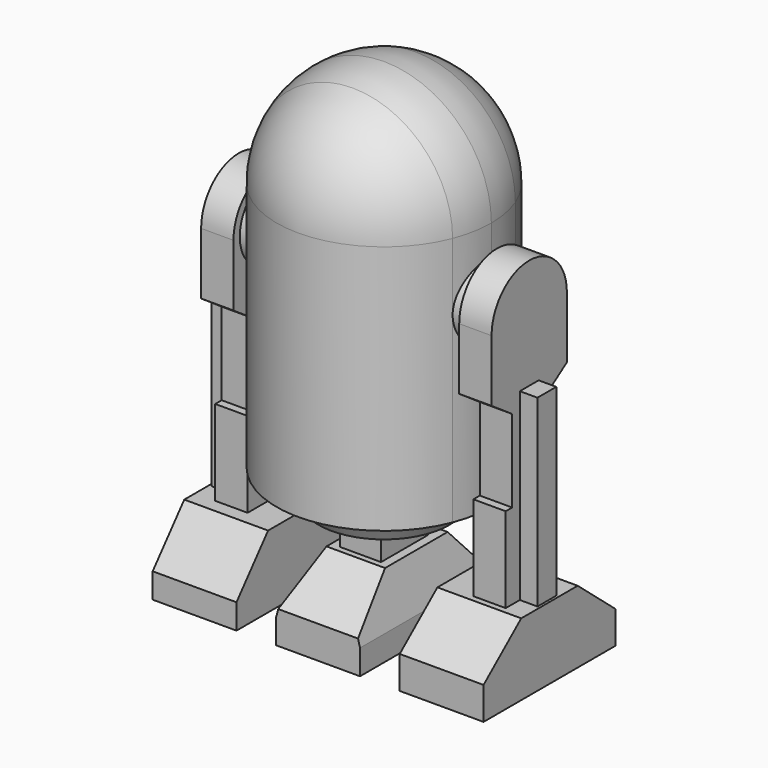
from build123d import *

# Parameters (mm, degrees)
F1_DEPTH       = 539.75
F2_ANGLE       = 180
F3_START       = -146.05
F3_DEPTH       = 568.325
F4_W           = 69.85
F4_H           = 101.6
F7_DEPTH       = 69.85
F8_W           = 50.8
F8_H           = 431.8
F9_DEPTH       = 38.1
F6_R           = 84.582
F11_DEPTH      = 627.0625
F12_R          = 177.8
F13_DEPTH      = 63.5
F14_SIZE2      = 36.661732
F14_SIZE       = 63.49999
F16_W          = 180.975
F16_H          = 355.6
F17_DEPTH      = 155.575
F18_W          = 88.9
F18_H          = 127
F19_DEPTH      = 76.2
F20_C1_SIZE2   = 85.2525225276
F20_C1_SIZE    = 101.6
F20_C2_SIZE2   = 85.2525225276
F20_C2_SIZE    = 101.6
F20_C3_SIZE2   = 85.2525225276
F20_C3_SIZE    = 101.6
F20_C4_SIZE2   = 85.2525225276
F20_C4_SIZE    = 101.6
F20_C5_SIZE2   = 101.6
F20_C5_SIZE    = 85.2525225276
F20_C6_SIZE2   = 85.2525225276
F20_C6_SIZE    = 101.6
F21_SIZE2      = 27.223637951
F21_SIZE       = 101.6
F21_2_SIZE2    = 27.223637951
F21_2_SIZE     = 101.6
F23_DEPTH      = 1136.65
F23_DEPTH_BACK = 101.6
F22_W          = 6.35
F22_H          = 457.2
F22_W_2        = 736.6
F22_H_2        = 6.35
F24_DEPTH      = 12.7
F25_DEPTH      = 1136.65
F26_W          = 38.1
F26_H          = 88.9
F27_DEPTH      = 457.2
F29_W          = 38.1
F29_H          = 63.5
F30_DEPTH      = 6.35
F31_W          = 38.1
F31_H          = 63.5
F32_DEPTH      = 12.7
F31_W_2        = 812.8
F31_H_2        = 114.3
F33_W          = 38.1
F33_H          = 584.2
F34_DEPTH      = 88.9
F35_W          = 38.1
F35_H          = 63.5
F36_DEPTH      = 736.6


# Not quite as in the source:
# - a fillet or chamfer is up to 0.001 mm smaller than in the source, because OpenCascade refuses the exact size
# - a feature of the source that left no trace in its solid (it failed there, or was rolled back) is left out


with BuildPart() as f1:
    # F0 (on Top) → F1 (new body)
    with BuildSketch(Plane.XY):
        with BuildLine():
            ThreePointArc((215.7904907567, -84.582), (227.743816184, -43.0395726621), (231.775, 0))
            ThreePointArc((231.775, 0), (227.743816184, 43.0395726621), (215.7904907567, 84.582))
            ThreePointArc((215.7904907567, 84.582), (130.6056231083, 191.4727704858), (0, 231.775))
            Line((0, 231.775), (0, 0))
            Line((0, 0), (0, -231.775))
            ThreePointArc((0, -231.775), (130.6056231083, -191.4727704858), (215.7904907567, -84.582))
        make_face()
        with BuildLine():
            Line((0, 0), (0, 231.775))
            ThreePointArc((0, 231.775), (-130.6056231083, 191.4727704858), (-215.7904907567, 84.582))
            ThreePointArc((-215.7904907567, 84.582), (-231.775, 0), (-215.7904907567, -84.582))
            ThreePointArc((-215.7904907567, -84.582), (-130.6056231083, -191.4727704858), (0, -231.775))
            Line((0, -231.775), (0, 0))
        make_face()
    extrude(amount=-F1_DEPTH)

    # F0 (on Top) → F2 (revolve)
    with BuildSketch(Plane.XY):
        with BuildLine():
            ThreePointArc((215.7904907567, -84.582), (227.743816184, -43.0395726621), (231.775, 0))
            ThreePointArc((231.775, 0), (227.743816184, 43.0395726621), (215.7904907567, 84.582))
            ThreePointArc((215.7904907567, 84.582), (130.6056231083, 191.4727704858), (0, 231.775))
            Line((0, 231.775), (0, 0))
            Line((0, 0), (0, -231.775))
            ThreePointArc((0, -231.775), (130.6056231083, -191.4727704858), (215.7904907567, -84.582))
        make_face()
    revolve(axis=Axis((0, -115.8875, 0), (0, -1, 0)), revolution_arc=F2_ANGLE)



with BuildPart() as f3:
    # F0 (on Top) → F3 (new body)
    with BuildSketch(Plane.XY.offset(F3_START)):
        Polygon((243.68125, 0), (243.68125, -84.582), (243.68125, -101.6), (313.53125, -101.6), (313.53125, -50.8), (313.53125, 0), align=None)
        Polygon((243.68125, 101.6), (243.68125, 84.582), (243.68125, 0), (313.53125, 0), (313.53125, 50.8), (313.53125, 101.6), align=None)
    extrude(amount=-F3_DEPTH)

    # F4 (on face) → F5 (revolve)
    with BuildSketch(Plane.XY.offset(-146.05)):
        with Locations((278.60625, -50.8)):
            Rectangle(F4_W, F4_H)
    revolve(axis=Axis((278.60625, 0, -146.05), (-1, 0, 0)))

    # F6 (on face) → F7 (cut, through all)
    with BuildSketch(Plane.YZ.offset(313.53125)):
        Polygon((101.6, -279.4), (46.0375, -317.5), (46.0375, -495.3), (63.5, -495.3), (63.5, -714.375), (101.6, -714.375), align=None)
        Polygon((-101.6, -714.375), (-63.5, -714.375), (-63.5, -495.3), (-46.0375, -495.3), (-46.0375, -317.5), (-101.6, -279.4), align=None)
    extrude(amount=-F7_DEPTH, mode=Mode.SUBTRACT)

    # F8 (on face) → F9 (join)
    with BuildSketch(Plane.YZ.offset(313.53125)):
        with Locations((0, -498.475)):
            Rectangle(F8_W, F8_H)
    extrude(amount=F9_DEPTH)


with BuildPart() as f10_1:
    # F10: instance of F3
    add(f3.part.mirror(Plane.YZ))


with BuildPart() as f1_1:
    add(f1.part)

    add(f3.part)  # F11 merges F3

    add(f10_1.part)  # F11 merges F10_1
    # F6 (on face) → F11 (join, through all)
    with BuildSketch(Plane.YZ.offset(313.53125)):
        with Locations((0, -146.05)):
            Circle(F6_R)
    extrude(amount=-F11_DEPTH)

    # F12 (on face) → F13 (join)
    with BuildSketch(Plane(origin=(0, 0, -539.75), x_dir=(1, 0, 0), z_dir=(0, 0, -1))):
        Circle(F12_R)
    extrude(amount=F13_DEPTH)

    # F14 (size 63.5 and 36.6617420935 in the source; OpenCascade refuses exactly that, so slightly less here)
    f14_edges = [f1_1.edges().sort_by_distance(p)[0] for p in [
        (-177.8, 0, -603.25),
    ]]
    f14_side = f1_1.faces().sort_by_distance((-177.8, 0, -571.5))[0]
    chamfer(f14_edges, length=F14_SIZE, length2=F14_SIZE2, reference=f14_side)

    # F16 (on offset) → F17, piece 2 (join)
    with BuildSketch(Plane.XY.offset(-835.025)):
        with Locations((-266.7, 0)):
            Rectangle(F16_W, F16_H)
        with Locations((266.7, 0)):
            Rectangle(F16_W, F16_H)
    extrude(amount=F17_DEPTH)



with BuildPart() as f17:
    # F16 (on offset) → F17 (new body)
    with BuildSketch(Plane.XY.offset(-835.025)):
        Rectangle(F16_W, F16_H)
    extrude(amount=F17_DEPTH)


with BuildPart() as f1_2:
    add(f1_1.part)

    add(f17.part)  # F19 merges F17
    # F18 (on face) → F19 (join, through all)
    with BuildSketch(Plane.XY.offset(-679.45)):
        Rectangle(F18_W, F18_H)
    extrude(amount=F19_DEPTH)

    # F20: chamfer of 101.6 x 85.2525225276 on 6 edges, made by hand

    # F20_c1
    f20_c1_edges = [f1_2.edges().sort_by_distance(p)[0] for p in [
        (0, 177.8, -679.45),
    ]]
    f20_c1_side = f1_2.faces().sort_by_distance((0, 177.8, -681.1550504506))[0]
    chamfer(f20_c1_edges, length=F20_C1_SIZE, length2=F20_C1_SIZE2, reference=f20_c1_side)

    # F20_c2
    f20_c2_edges = [f1_2.edges().sort_by_distance(p)[0] for p in [
        (0, -177.8, -679.45),
    ]]
    f20_c2_side = f1_2.faces().sort_by_distance((0, -176.0949495494, -679.45))[0]
    chamfer(f20_c2_edges, length=F20_C2_SIZE, length2=F20_C2_SIZE2, reference=f20_c2_side)

    # F20_c3
    f20_c3_edges = [f1_2.edges().sort_by_distance(p)[0] for p in [
        (266.7, 177.8, -679.45),
    ]]
    f20_c3_side = f1_2.faces().sort_by_distance((266.7, 176.0949495494, -679.45))[0]
    chamfer(f20_c3_edges, length=F20_C3_SIZE, length2=F20_C3_SIZE2, reference=f20_c3_side)

    # F20_c4
    f20_c4_edges = [f1_2.edges().sort_by_distance(p)[0] for p in [
        (266.7, -177.8, -679.45),
    ]]
    f20_c4_side = f1_2.faces().sort_by_distance((266.7, -176.0949495494, -679.45))[0]
    chamfer(f20_c4_edges, length=F20_C4_SIZE, length2=F20_C4_SIZE2, reference=f20_c4_side)

    # F20_c5
    f20_c5_edges = [f1_2.edges().sort_by_distance(p)[0] for p in [
        (-266.7, -177.8, -679.45),
    ]]
    f20_c5_side = f1_2.faces().sort_by_distance((-266.7, -176.0949495494, -679.45))[0]
    chamfer(f20_c5_edges, length=F20_C5_SIZE, length2=F20_C5_SIZE2, reference=f20_c5_side)

    # F20_c6
    f20_c6_edges = [f1_2.edges().sort_by_distance(p)[0] for p in [
        (-266.7, 177.8, -679.45),
    ]]
    f20_c6_side = f1_2.faces().sort_by_distance((-266.7, 176.0949495494, -679.45))[0]
    chamfer(f20_c6_edges, length=F20_C6_SIZE, length2=F20_C6_SIZE2, reference=f20_c6_side)

    # F21
    f21_edges = [f1_2.edges().sort_by_distance(p)[0] for p in [
        (-90.4875, 8.173739, -679.45),
    ]]
    f21_side = f1_2.faces().sort_by_distance((-90.4875, -0.505764, -765.896297))[0]
    chamfer(f21_edges, length=F21_SIZE, length2=F21_SIZE2, reference=f21_side)

    # F21#2
    f21_2_edges = [f1_2.edges().sort_by_distance(p)[0] for p in [
        (90.4875, 8.173739, -679.45),
    ]]
    f21_2_side = f1_2.faces().sort_by_distance((90.4875, -0.505764, -765.896297))[0]
    chamfer(f21_2_edges, length=F21_2_SIZE, length2=F21_2_SIZE2, reference=f21_2_side)


with BuildPart() as f23:
    # F22 (on offset) → F23 (new body, two sides)
    with BuildSketch(Plane.XY.offset(-835.025)) as f23_sk:
        Polygon((400.05, 228.6), (406.4, 228.6), (406.4, 292.1), (368.3, 292.1), (368.3, 285.75), (368.3, 228.6), align=None)
    extrude(amount=F23_DEPTH)
    extrude(f23_sk.sketch, amount=-F23_DEPTH_BACK)


with BuildPart() as f23b:
    # F22 (on offset) → F23, piece 2 (new body, two sides)
    with BuildSketch(Plane.XY.offset(-835.025)) as f23_2_sk:
        Polygon((368.3, -292.1), (406.4, -292.1), (406.4, -228.6), (400.05, -228.6), (368.3, -228.6), (368.3, -285.75), align=None)
    extrude(amount=F23_DEPTH)
    extrude(f23_2_sk.sketch, amount=-F23_DEPTH_BACK)


with BuildPart() as f23c:
    # F22 (on offset) → F23, piece 3 (new body, two sides)
    with BuildSketch(Plane.XY.offset(-835.025)) as f23_3_sk:
        Polygon((-406.4, 292.1), (-406.4, 228.6), (-400.05, 228.6), (-368.3, 228.6), (-368.3, 285.75), (-368.3, 292.1), align=None)
    extrude(amount=F23_DEPTH)
    extrude(f23_3_sk.sketch, amount=-F23_DEPTH_BACK)


with BuildPart() as f23d:
    # F22 (on offset) → F23, piece 4 (new body, two sides)
    with BuildSketch(Plane.XY.offset(-835.025)) as f23_4_sk:
        Polygon((-406.4, -292.1), (-368.3, -292.1), (-368.3, -285.75), (-368.3, -228.6), (-400.05, -228.6), (-406.4, -228.6), align=None)
    extrude(amount=F23_DEPTH)
    extrude(f23_4_sk.sketch, amount=-F23_DEPTH_BACK)


with BuildPart() as f24:
    # F22 (on offset) → F24 (new body)
    with BuildSketch(Plane.XY.offset(-835.025)):
        with Locations((-403.225, 0)):
            Rectangle(F22_W, F22_H)
        Polygon((-368.3, -285.75), (368.3, -285.75), (368.3, -228.6), (400.05, -228.6), (400.05, 228.6), (368.3, 228.6), (368.3, 285.75), (-368.3, 285.75), (-368.3, 228.6), (-400.05, 228.6), (-400.05, -228.6), (-368.3, -228.6), align=None)
        with Locations((0, 288.925)):
            Rectangle(F22_W_2, F22_H_2)
        with Locations((0, -288.925)):
            Rectangle(F22_W_2, F22_H_2)
        with Locations((403.225, 0)):
            Rectangle(F22_W, F22_H)
    extrude(amount=-F24_DEPTH)


with BuildPart() as f25:
    # F22 (on offset) → F25 (new body, through all)
    with BuildSketch(Plane.XY.offset(-835.025)):
        with Locations((0, 288.925)):
            Rectangle(F22_W_2, F22_H_2)
    extrude(amount=F25_DEPTH)


with BuildPart() as f25b:
    # F22 (on offset) → F25, piece 2 (new body, through all)
    with BuildSketch(Plane.XY.offset(-835.025)):
        with Locations((403.225, 0)):
            Rectangle(F22_W, F22_H)
    extrude(amount=F25_DEPTH)


with BuildPart() as f25c:
    # F22 (on offset) → F25, piece 3 (new body, through all)
    with BuildSketch(Plane.XY.offset(-835.025)):
        with Locations((0, -288.925)):
            Rectangle(F22_W_2, F22_H_2)
    extrude(amount=F25_DEPTH)


with BuildPart() as f25d:
    # F22 (on offset) → F25, piece 4 (new body, through all)
    with BuildSketch(Plane.XY.offset(-835.025)):
        with Locations((-403.225, 0)):
            Rectangle(F22_W, F22_H)
    extrude(amount=F25_DEPTH)


with BuildPart() as f27:
    # F26 (on face) → F27 (new body, through all)
    with BuildSketch(Plane(origin=(0, -228.6, 0), x_dir=(-1, 0, 0), z_dir=(0, 1, 0))):
        with Locations((-387.35, -892.175)):
            Rectangle(F26_W, F26_H)
    extrude(amount=F27_DEPTH)


with BuildPart() as f28_1:
    # F28: instance of F27
    add(f27.part.mirror(Plane.YZ))


with BuildPart() as f30:
    # F29 (on face) → F30 (new body)
    with BuildSketch(Plane.XY.offset(301.625)):
        Polygon((368.3, 228.6), (368.3, 292.1), (-406.4, 292.1), (-406.4, -292.1), (406.4, -292.1), (406.4, 228.6), align=None)
        with Locations((387.35, 260.35)):
            Rectangle(F29_W, F29_H)
    extrude(amount=F30_DEPTH)


with BuildPart() as f32:
    # F31 (on face) → F32 (new body)
    with BuildSketch(Plane(origin=(0, 0, -936.625), x_dir=(1, 0, 0), z_dir=(0, 0, -1))):
        Polygon((-406.4, -177.8), (-406.4, -292.1), (368.3, -292.1), (368.3, -228.6), (406.4, -228.6), (406.4, -177.8), align=None)
        with Locations((387.35, -260.35)):
            Rectangle(F31_W, F31_H)
    extrude(amount=F32_DEPTH)


with BuildPart() as f32b:
    # F31 (on face) → F32, piece 2 (new body)
    with BuildSketch(Plane(origin=(0, 0, -936.625), x_dir=(1, 0, 0), z_dir=(0, 0, -1))):
        with Locations((0, 234.95)):
            Rectangle(F31_W_2, F31_H_2)
    extrude(amount=F32_DEPTH)


with BuildPart() as f34:
    # F33 (on face) → F34 (new body, through all)
    with BuildSketch(Plane(origin=(0, 0, -847.725), x_dir=(1, 0, 0), z_dir=(0, 0, -1))):
        with Locations((57.15, 0)):
            Rectangle(F33_W, F33_H)
    extrude(amount=F34_DEPTH)


with BuildPart() as f34b:
    # F33 (on face) → F34, piece 2 (new body, through all)
    with BuildSketch(Plane(origin=(0, 0, -847.725), x_dir=(1, 0, 0), z_dir=(0, 0, -1))):
        with Locations((-57.15, 0)):
            Rectangle(F33_W, F33_H)
    extrude(amount=F34_DEPTH)


with BuildPart() as f36:
    # F35 (on face) → F36 (new body, through all)
    with BuildSketch(Plane(origin=(368.3, 0, 0), x_dir=(0, -1, 0), z_dir=(-1, 0, 0))):
        with Locations((-266.7, -803.275)):
            Rectangle(F35_W, F35_H)
    extrude(amount=F36_DEPTH)


solid = f1_2.part
